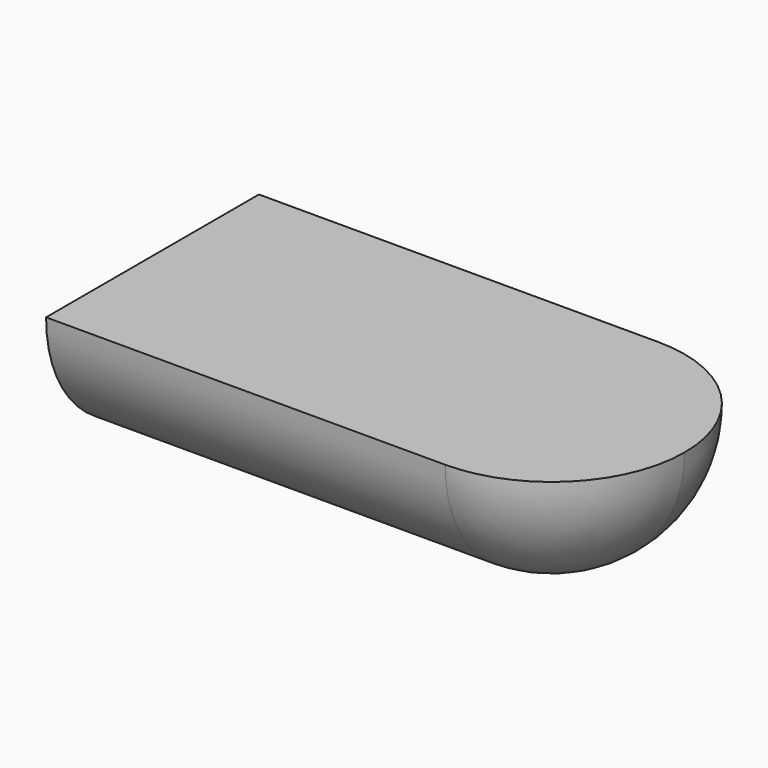
from build123d import *

# Parameters (mm, degrees)
F0_W     = 76.2
F0_H     = 25.4
F1_DEPTH = 50.8
F2_R     = 25.39999
F3_R     = 25.39999


# Not quite as in the source:
# - a fillet or chamfer is up to 0.001 mm smaller than in the source, because OpenCascade refuses the exact size


with BuildPart() as f1:
    # F0 (on Front) → F1 (new body)
    with BuildSketch(Plane.XZ):
        with Locations((21.0978503615, -17.8415966735)):
            Rectangle(F0_W, F0_H)
        with BuildLine():
            Line((84.5978503615, -5.1415966735), (59.1978503615, -5.1415966735))
            Line((59.1978503615, -5.1415966735), (59.1978503615, -30.5415966735))
            ThreePointArc((59.1978503615, -30.5415966735), (77.1583626036, -23.1021089156), (84.5978503615, -5.1415966735))
        make_face()
    extrude(amount=F1_DEPTH)

    # F2 (radius 25.4 in the source; OpenCascade refuses exactly that, so slightly less here)
    f2_edges = [f1.edges().sort_by_distance(p)[0] for p in [
        (21.09785, -50.8, -30.541597),
    ]]
    fillet(f2_edges, radius=F2_R)

    # F3 (radius 25.4 in the source; OpenCascade refuses exactly that, so slightly less here)
    f3_edges = [f1.edges().sort_by_distance(p)[0] for p in [
        (21.09785, 0, -30.541597),
    ]]
    fillet(f3_edges, radius=F3_R)


solid = f1.part
